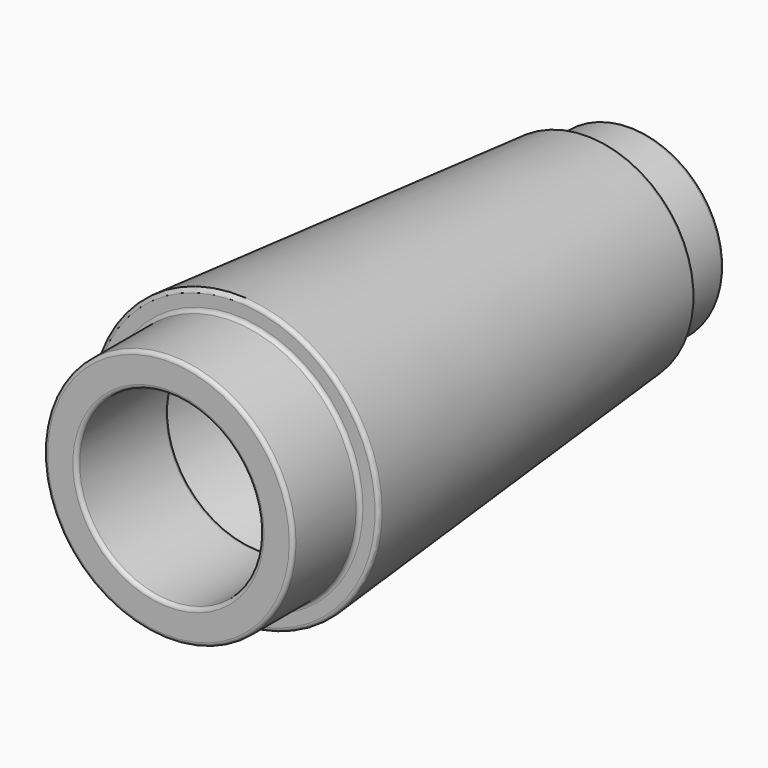
from build123d import *

# Parameters (mm, degrees)
F0_R       = 3.795
F1_DEPTH   = 11.6
F2_R       = 2.81
F1_FACE1_R = 3.795
F4_R       = 2.44
F5_DEPTH   = 1.41
F6_R       = 3.27
F7_DEPTH   = 2.17
F8_T       = -0.86
F9_R       = 0.1


with BuildPart() as f1:
    # F0 (on Front) → F1 (new body)
    with BuildSketch(Plane.XZ):
        Circle(F0_R)
    extrude(amount=-F1_DEPTH)

    # F2 (on face) → F3 section 0
    with BuildSketch(Plane(origin=(0, 11.6, 0), x_dir=(-1, 0, 0), z_dir=(0, 1, 0))):
        Circle(F2_R)
    # F1_face1 (on face) → F3 section 1
    with BuildSketch(Plane.XZ):
        Circle(F1_FACE1_R)
    loft(mode=Mode.INTERSECT)

    # F4 (on face) → F5 (join)
    with BuildSketch(Plane(origin=(0, 11.6, 0), x_dir=(-1, 0, 0), z_dir=(0, 1, 0))):
        Circle(F4_R)
    extrude(amount=F5_DEPTH)

    # F6 (on face) → F7 (join)
    with BuildSketch(Plane.XZ):
        Circle(F6_R)
    extrude(amount=F7_DEPTH)

    # F8
    f8_openings = [f1.faces().sort_by_distance(p)[0] for p in [
        (0, 13.01, 0),
        (0, -2.17, 0),
    ]]
    offset(amount=F8_T, openings=f8_openings, kind=Kind.INTERSECTION)

    # F9
    f9_edges = [f1.edges().sort_by_distance(p)[0] for p in [
        (-3.27, 0, 0),
        (2.81, 11.6, 0),
        (-3.27, -2.17, 0),
        (3.795, 0, 0),
        (2.44, 13.01, 0),
        (-2.41, 0.86, 0),
        (-2.41, -2.17, 0),
        (2.44, 11.6, 0),
        (2.858879, 0.86, 0),
        (1.58, 13.01, 0),
        (1.58, 10.74, 0),
        (2.019931, 10.74, 0),
    ]]
    fillet(f9_edges, radius=F9_R)


solid = f1.part
